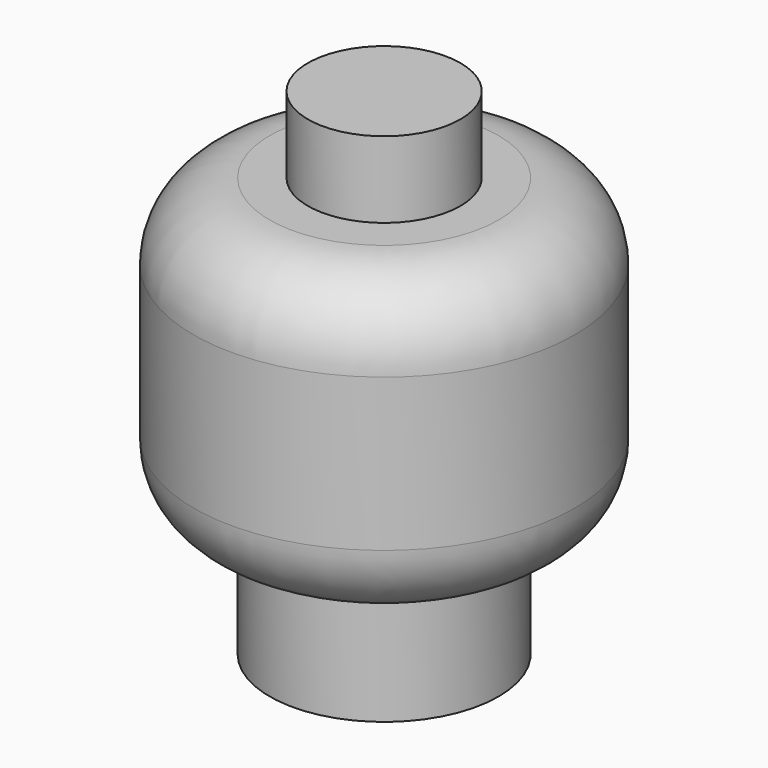
from build123d import *

# Parameters (mm, degrees)
F0_R     = 3
F1_DEPTH = 3
F2_R     = 5
F3_DEPTH = 8
F4_R     = 2
F5_DEPTH = 2
F6_R     = 1.99999
F7_R     = 2.5
F8_DEPTH = 8


# Not quite as in the source:
# - a fillet or chamfer is up to 0.001 mm smaller than in the source, because OpenCascade refuses the exact size


with BuildPart() as f1:
    # F0 (on Top) → F1 (new body)
    with BuildSketch(Plane.XY):
        Circle(F0_R)
    extrude(amount=F1_DEPTH)

    # F2 (on face) → F3 (join)
    with BuildSketch(Plane.XY.offset(3)):
        Circle(F2_R)
    extrude(amount=F3_DEPTH)

    # F4 (on face) → F5 (join)
    with BuildSketch(Plane.XY.offset(11)):
        Circle(F4_R)
    extrude(amount=F5_DEPTH)

    # F6 (radius 2 in the source; OpenCascade refuses exactly that, so slightly less here)
    f6_edges = [f1.edges().sort_by_distance(p)[0] for p in [
        (-5, 0, 11),
        (-5, 0, 3),
    ]]
    fillet(f6_edges, radius=F6_R)

    # F7 (on face) → F8 (cut)
    with BuildSketch(Plane(origin=(0, 0, 0), x_dir=(1, 0, 0), z_dir=(0, 0, -1))):
        Circle(F7_R)
    extrude(amount=-F8_DEPTH, mode=Mode.SUBTRACT)


solid = f1.part
